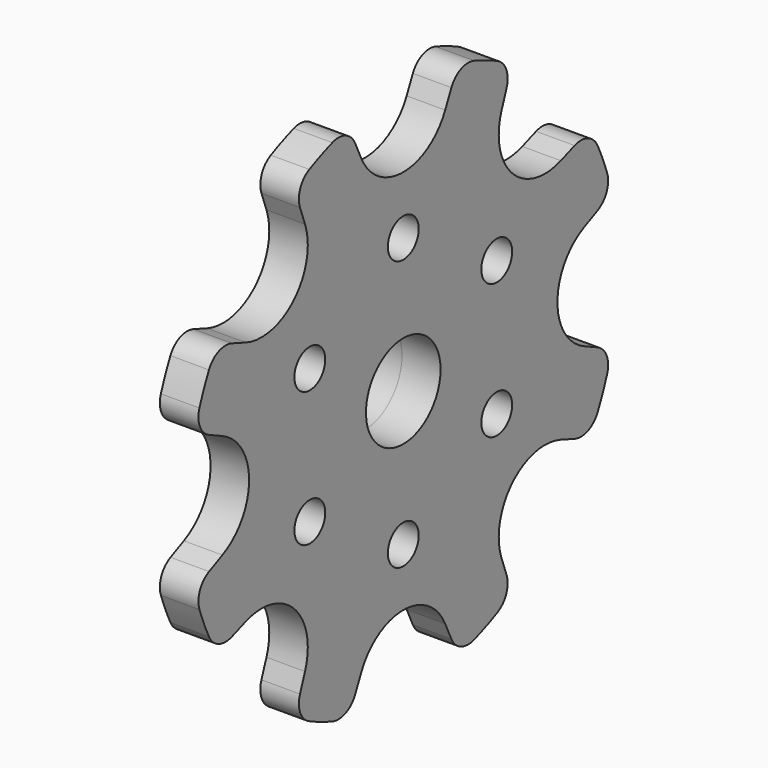
from build123d import *
from build123d import SkipClean  # not in build123d's __all__

# Parameters (mm, degrees)
F0_R     = 2.5
F0_R_2   = 6.05
F1_DEPTH = 5
F2_W     = 7
F2_H     = 5


with BuildPart() as f1:
    # F0 (on Right) → F1 (new body)
    with BuildSketch(Plane.YZ):
        with BuildLine():
            ThreePointArc((6.7973084028, 29.3303630369), (0, 25), (-6.7973084028, 29.3303630369))
            Line((-6.7973084028, 29.3303630369), (-7.8035829138, 31.4883256898))
            ThreePointArc((-7.8035829138, 31.4883256898), (-9.3550783484, 32.9840034331), (-11.5089912382, 33.0536400519))
            ThreePointArc((-11.5089912382, 33.0536400519), (-13.3939201328, 32.3357836379), (-15.2343672744, 31.5105387727))
            ThreePointArc((-15.2343672744, 31.5105387727), (-16.7081731596, 29.9382518369), (-16.7476422276, 27.7835750194))
            Line((-16.7476422276, 27.7835750194), (-15.9332757327, 25.5461214635))
            ThreePointArc((-15.9332757327, 25.5461214635), (-17.6776695297, 17.6776695297), (-25.5461214635, 15.9332757327))
            Line((-25.5461214635, 15.9332757327), (-27.7835750194, 16.7476422276))
            ThreePointArc((-27.7835750194, 16.7476422276), (-29.9382518369, 16.7081731596), (-31.5105387727, 15.2343672744))
            ThreePointArc((-31.5105387727, 15.2343672744), (-32.3357836379, 13.3939201328), (-33.0536400519, 11.5089912382))
            ThreePointArc((-33.0536400519, 11.5089912382), (-32.9840034331, 9.3550783484), (-31.4883256898, 7.8035829138))
            Line((-31.4883256898, 7.8035829138), (-29.3303630369, 6.7973084028))
            ThreePointArc((-29.3303630369, 6.7973084028), (-25, 0), (-29.3303630369, -6.7973084028))
            Line((-29.3303630369, -6.7973084028), (-31.4883256898, -7.8035829138))
            ThreePointArc((-31.4883256898, -7.8035829138), (-32.9840034331, -9.3550783484), (-33.0536400519, -11.5089912382))
            ThreePointArc((-33.0536400519, -11.5089912382), (-32.3357836379, -13.3939201328), (-31.5105387727, -15.2343672744))
            ThreePointArc((-31.5105387727, -15.2343672744), (-29.9382518369, -16.7081731596), (-27.7835750194, -16.7476422276))
            Line((-27.7835750194, -16.7476422276), (-25.5461214635, -15.9332757327))
            ThreePointArc((-25.5461214635, -15.9332757327), (-17.6776695297, -17.6776695297), (-15.9332757327, -25.5461214635))
            Line((-15.9332757327, -25.5461214635), (-16.7476422276, -27.7835750194))
            ThreePointArc((-16.7476422276, -27.7835750194), (-16.7081731596, -29.9382518369), (-15.2343672744, -31.5105387727))
            ThreePointArc((-15.2343672744, -31.5105387727), (-13.3939201328, -32.3357836379), (-11.5089912382, -33.0536400519))
            ThreePointArc((-11.5089912382, -33.0536400519), (-9.3550783484, -32.9840034331), (-7.8035829138, -31.4883256898))
            Line((-7.8035829138, -31.4883256898), (-6.7973084028, -29.3303630369))
            ThreePointArc((-6.7973084028, -29.3303630369), (0, -25), (6.7973084028, -29.3303630369))
            Line((6.7973084028, -29.3303630369), (7.8035829138, -31.4883256898))
            ThreePointArc((7.8035829138, -31.4883256898), (9.3550783484, -32.9840034331), (11.5089912382, -33.0536400519))
            ThreePointArc((11.5089912382, -33.0536400519), (13.3939201328, -32.3357836379), (15.2343672744, -31.5105387727))
            ThreePointArc((15.2343672744, -31.5105387727), (16.7081731596, -29.9382518369), (16.7476422276, -27.7835750194))
            Line((16.7476422276, -27.7835750194), (15.9332757327, -25.5461214635))
            ThreePointArc((15.9332757327, -25.5461214635), (17.6776695297, -17.6776695297), (25.5461214635, -15.9332757327))
            Line((25.5461214635, -15.9332757327), (27.7835750194, -16.7476422276))
            ThreePointArc((27.7835750194, -16.7476422276), (29.9382518369, -16.7081731596), (31.5105387727, -15.2343672744))
            ThreePointArc((31.5105387727, -15.2343672744), (32.3357836379, -13.3939201328), (33.0536400519, -11.5089912382))
            ThreePointArc((33.0536400519, -11.5089912382), (32.9840034331, -9.3550783484), (31.4883256898, -7.8035829138))
            Line((31.4883256898, -7.8035829138), (29.3303630369, -6.7973084028))
            ThreePointArc((29.3303630369, -6.7973084028), (25, 0), (29.3303630369, 6.7973084028))
            Line((29.3303630369, 6.7973084028), (31.4883256898, 7.8035829138))
            ThreePointArc((31.4883256898, 7.8035829138), (32.9840034331, 9.3550783484), (33.0536400519, 11.5089912382))
            ThreePointArc((33.0536400519, 11.5089912382), (32.3357836379, 13.3939201328), (31.5105387727, 15.2343672744))
            ThreePointArc((31.5105387727, 15.2343672744), (29.9382518369, 16.7081731596), (27.7835750194, 16.7476422276))
            Line((27.7835750194, 16.7476422276), (25.5461214635, 15.9332757327))
            ThreePointArc((25.5461214635, 15.9332757327), (17.6776695297, 17.6776695297), (15.9332757327, 25.5461214635))
            Line((15.9332757327, 25.5461214635), (16.7476422276, 27.7835750194))
            ThreePointArc((16.7476422276, 27.7835750194), (16.7081731596, 29.9382518369), (15.2343672744, 31.5105387727))
            ThreePointArc((15.2343672744, 31.5105387727), (13.3939201328, 32.3357836379), (11.5089912382, 33.0536400519))
            ThreePointArc((11.5089912382, 33.0536400519), (9.3550783484, 32.9840034331), (7.8035829138, 31.4883256898))
            Line((7.8035829138, 31.4883256898), (6.7973084028, 29.3303630369))
        make_face()
        with Locations((-15.1554445662, -8.75)):
            Circle(F0_R, mode=Mode.SUBTRACT)
        with Locations((0, -17.5)):
            Circle(F0_R, mode=Mode.SUBTRACT)
        with Locations((15.1554445662, -8.75)):
            Circle(F0_R, mode=Mode.SUBTRACT)
        with Locations((-15.1554445662, 8.75)):
            Circle(F0_R, mode=Mode.SUBTRACT)
        Circle(F0_R_2, mode=Mode.SUBTRACT)
        with Locations((15.1554445662, 8.75)):
            Circle(F0_R, mode=Mode.SUBTRACT)
        with Locations((0, 17.5)):
            Circle(F0_R, mode=Mode.SUBTRACT)
    extrude(amount=F1_DEPTH)

    # F2 (on Front) → F3 (revolve)
    with BuildSketch(Plane.XZ):
        with Locations((-3.5, 8.55)):
            Rectangle(F2_W, F2_H)
    with SkipClean():  # cleaning this boolean's faces spoils the solid; the shape is the same uncleaned
        revolve(axis=Axis((9.7608398646, 0, 0), (1, 0, 0)))


solid = f1.part
